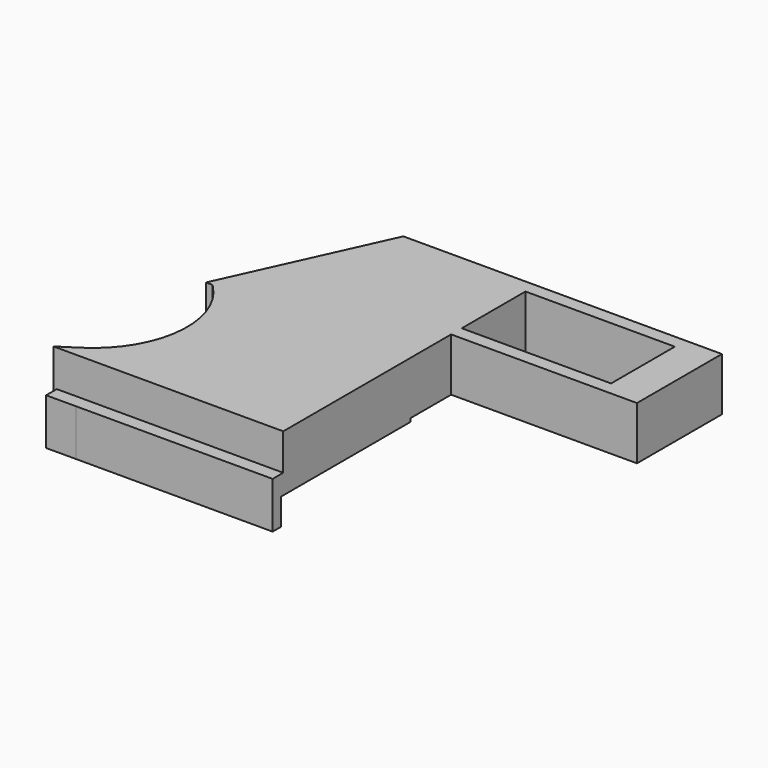
from build123d import *

# Parameters (mm, degrees)
F0_W     = 22.5
F0_H     = 12
F0_W_2   = 16.6362704164
F0_H_2   = 1.4672726393
F1_DEPTH = 8.5
F0_W_3   = 12.9140389063
F0_H_3   = 0.4558046321
F0_H_4   = 1.5437308085
F2_DEPTH = 3
F3_DEPTH = 4
F4_DEPTH = 0.5
F5_DEPTH = 0.5
F6_DEPTH = 4


# Not quite as in the source:
# - a feature names something its author has since deleted; it is built from what else it names


with BuildPart() as f1:
    # F0 (on Top) → F1 (new body)
    with BuildSketch(Plane.XY):
        Polygon((-28.1854607165, -113.3383650622), (-15.2103829287, -113.3383650622), (-15.2103829287, -112.8061022609), (-15.2103829287, -111.3388296217), (-15.2103829287, -105.6495462671), (-21.261529997, -105.6495462671), (-21.261529997, -89.6495462671), (-35.2103829287, -89.6495462671), (-46.0062867338, -113.3383650622), (-45.0214308559, -113.3383650622), (-44.8217311329, -113.3383650622), (-44.8217311329, -112.8061022609), (-44.8217311329, -111.3388296217), (-28.1854607165, -111.3388296217), (-28.1854607165, -112.8061022609), align=None)
        Polygon((-28.1244218349, -137.2695039054), (-15.2103829287, -137.2695039054), (-15.2103829287, -136.6045172354), (-15.2103829287, -114.0332519535), (-15.2103829287, -113.3383650622), (-28.1854607165, -113.3383650622), (-35.2103829287, -113.3383650622), (-35.2103829287, -125.3039344838), (-35.2103829287, -137.2695039054), align=None)
        with BuildLine():
            Line((-49.3365414441, -137.2695039054), (-35.2103829287, -137.2695039054))
            Line((-35.2103829287, -137.2695039054), (-35.2103829287, -125.3039344838))
            Line((-35.2103829287, -125.3039344838), (-35.2103829287, -113.3383650622))
            Line((-35.2103829287, -113.3383650622), (-44.8217311329, -113.3383650622))
            Line((-44.8217311329, -113.3383650622), (-44.8217311329, -113.5371806076))
            ThreePointArc((-44.8217311329, -113.5371806076), (-40.72117222, -125.1132769851), (-47.1813260123, -135.5577493852))
            Line((-47.1813260123, -135.5577493852), (-49.8537484313, -137.2695039054))
            Line((-49.8537484313, -137.2695039054), (-49.3365414441, -137.2695039054))
        make_face()
        Polygon((-21.261529997, -105.6495462671), (-15.2103829287, -105.6495462671), (7.2896170713, -105.6495462671), (12.7896170713, -105.6495462671), (12.7896170713, -91.6495462671), (12.7896170713, -89.6495462671), (-15.2103829287, -89.6495462671), (-21.261529997, -89.6495462671), align=None)
        with Locations((-3.9603829287, -97.6495462671)):
            Rectangle(F0_W, F0_H, mode=Mode.SUBTRACT)
        Polygon((-35.2103829287, -113.3383650622), (-28.1854607165, -113.3383650622), (-28.1854607165, -112.8061022609), (-44.8217311329, -112.8061022609), (-44.8217311329, -113.3383650622), align=None)
        with Locations((-36.5035959247, -112.0724659413)):
            Rectangle(F0_W_2, F0_H_2)
        Polygon((-44.8217311329, -113.5371806076), (-44.8217311329, -113.3383650622), (-45.0214308559, -113.3383650622), align=None)
    extrude(amount=F1_DEPTH)

    # F0 (on Top) → F2 (join)
    with BuildSketch(Plane.XY):
        Polygon((-28.1244218349, -137.7253085375), (-28.1244218349, -137.2695039054), (-35.2103829287, -137.2695039054), (-49.3365414441, -137.2695039054), (-49.3365414441, -137.7253085375), align=None)
        Polygon((-28.1244218349, -139.269039346), (-28.1244218349, -137.7253085375), (-49.3365414441, -137.7253085375), (-49.3365414441, -139.2803862691), (-44.8217311329, -139.269039346), align=None)
        with Locations((-21.6674023818, -137.4974062214)):
            Rectangle(F0_W_3, F0_H_3)
        with Locations((-21.6674023818, -138.4971739417)):
            Rectangle(F0_W_3, F0_H_4)
    extrude(amount=F2_DEPTH)

    # F0 (on Top) → F3 (join)
    with BuildSketch(Plane.XY):
        Polygon((-28.1244218349, -139.269039346), (-28.1244218349, -137.7253085375), (-49.3365414441, -137.7253085375), (-49.3365414441, -139.2803862691), (-44.8217311329, -139.269039346), align=None)
        with Locations((-21.6674023818, -138.4971739417)):
            Rectangle(F0_W_3, F0_H_4)
    extrude(amount=-F3_DEPTH)

    # F0 (on Top) → F4 (cut)
    with BuildSketch(Plane.XY):
        Polygon((-28.1854607165, -113.3383650622), (-15.2103829287, -113.3383650622), (-15.2103829287, -112.8061022609), (-15.2103829287, -111.3388296217), (-15.2103829287, -105.6495462671), (-21.261529997, -105.6495462671), (-21.261529997, -89.6495462671), (-35.2103829287, -89.6495462671), (-46.0062867338, -113.3383650622), (-45.0214308559, -113.3383650622), (-44.8217311329, -113.3383650622), (-44.8217311329, -112.8061022609), (-44.8217311329, -111.3388296217), (-28.1854607165, -111.3388296217), (-28.1854607165, -112.8061022609), align=None)
        Polygon((-21.261529997, -105.6495462671), (-15.2103829287, -105.6495462671), (7.2896170713, -105.6495462671), (12.7896170713, -105.6495462671), (12.7896170713, -91.6495462671), (12.7896170713, -89.6495462671), (-15.2103829287, -89.6495462671), (-21.261529997, -89.6495462671), align=None)
        with Locations((-3.9603829287, -97.6495462671)):
            Rectangle(F0_W, F0_H, mode=Mode.SUBTRACT)
    extrude(amount=F4_DEPTH, mode=Mode.SUBTRACT)

    # F0 (on Top) → F5 (join)
    with BuildSketch(Plane.XY):
        with Locations((-36.5035959247, -112.0724659413)):
            Rectangle(F0_W_2, F0_H_2)
        Polygon((-35.2103829287, -113.3383650622), (-28.1854607165, -113.3383650622), (-28.1854607165, -112.8061022609), (-44.8217311329, -112.8061022609), (-44.8217311329, -113.3383650622), align=None)
    extrude(amount=F5_DEPTH)

    # F0 (on Top) → F6 (join)
    with BuildSketch(Plane.XY):
        with Locations((-36.5035959247, -112.0724659413)):
            Rectangle(F0_W_2, F0_H_2)
    extrude(amount=-F6_DEPTH)


solid = f1.part
